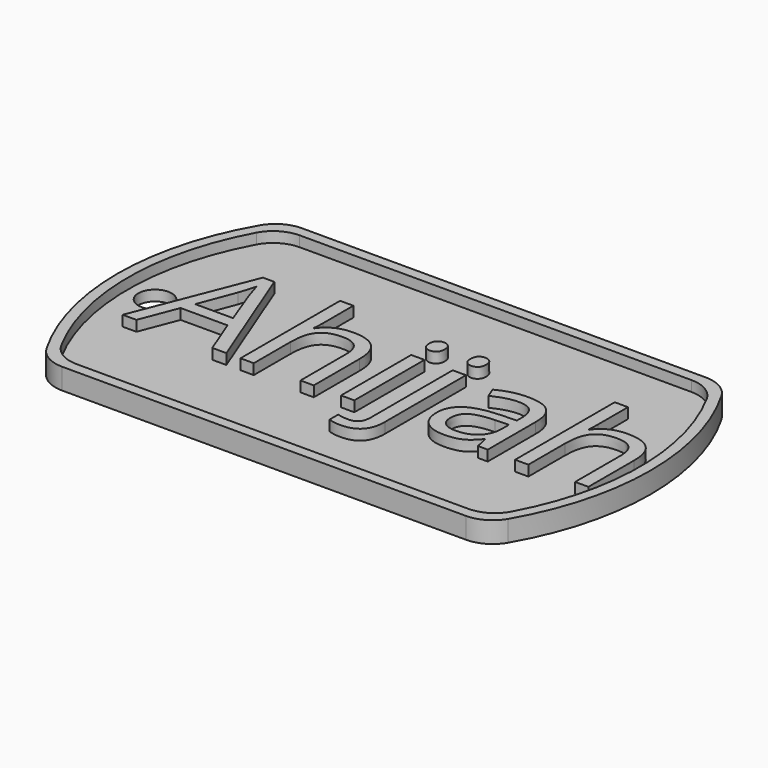
from build123d import *

# Parameters (mm, degrees)
F1_DEPTH     = 1
F3_DEPTH     = 1
F4_R         = 1.5875
F5_DEPTH     = 1
F6_TEXT_SIZE = 15.6169550286
F7_DEPTH     = 1


# Not quite as in the source:
# - Text() gives the source's letters only with a copy of the font that has no kerning and outlines rounded to 1/6400 em; it was checked with that copy


with BuildPart() as f1:
    # F0 (on Top) → F1 (new body)
    with BuildSketch(Plane.XY):
        with BuildLine():
            ThreePointArc((-19.2474145991, 14.2875), (-20.8349145991, 13.862130657), (-21.9970452561, 12.7))
            ThreePointArc((-21.9970452561, 12.7), (-25.4, 0), (-21.9970452561, -12.7))
            ThreePointArc((-21.9970452561, -12.7), (-20.8349145991, -13.862130657), (-19.2474145991, -14.2875))
            Line((-19.2474145991, -14.2875), (19.2474145991, -14.2875))
            ThreePointArc((19.2474145991, -14.2875), (20.8349145991, -13.862130657), (21.9970452561, -12.7))
            ThreePointArc((21.9970452561, -12.7), (25.4, 0), (21.9970452561, 12.7))
            ThreePointArc((21.9970452561, 12.7), (20.8349145991, 13.862130657), (19.2474145991, 14.2875))
            Line((19.2474145991, 14.2875), (-19.2474145991, 14.2875))
        make_face()
    extrude(amount=F1_DEPTH)

    # F2 (on face) → F3 (join)
    with BuildSketch(Plane.XY.offset(1)):
        with BuildLine():
            Line((19.2474145991, 14.2875), (-19.2474145991, 14.2875))
            ThreePointArc((-19.2474145991, 14.2875), (-20.8349145991, 13.862130657), (-21.9970452561, 12.7))
            ThreePointArc((-21.9970452561, 12.7), (-25.4, 0), (-21.9970452561, -12.7))
            ThreePointArc((-21.9970452561, -12.7), (-20.8349145991, -13.862130657), (-19.2474145991, -14.2875))
            Line((-19.2474145991, -14.2875), (19.2474145991, -14.2875))
            ThreePointArc((19.2474145991, -14.2875), (20.8349145991, -13.862130657), (21.9970452561, -12.7))
            ThreePointArc((21.9970452561, -12.7), (25.4, 0), (21.9970452561, 12.7))
            ThreePointArc((21.9970452561, 12.7), (20.8349145991, 13.862130657), (19.2474145991, 14.2875))
        make_face()
        with BuildLine():
            ThreePointArc((-21.4526124879, 11.6252061249), (-20.2856017842, 12.8404540819), (-18.6611352482, 13.2875))
            Line((-18.6611352482, 13.2875), (18.6611352482, 13.2875))
            ThreePointArc((18.6611352482, 13.2875), (20.2856017842, 12.8404540819), (21.4526124879, 11.6252061249))
            ThreePointArc((21.4526124879, 11.6252061249), (24.4, 0), (21.4526124879, -11.6252061249))
            ThreePointArc((21.4526124879, -11.6252061249), (20.2856017842, -12.8404540819), (18.6611352482, -13.2875))
            Line((18.6611352482, -13.2875), (-18.6611352482, -13.2875))
            ThreePointArc((-18.6611352482, -13.2875), (-20.2856017842, -12.8404540819), (-21.4526124879, -11.6252061249))
            ThreePointArc((-21.4526124879, -11.6252061249), (-24.4, 0), (-21.4526124879, 11.6252061249))
        make_face(mode=Mode.SUBTRACT)
    extrude(amount=F3_DEPTH)

    # F4 (on face) → F5 (cut)
    with BuildSketch(Plane.XY.offset(1)):
        with Locations((-21.821282804, 0)):
            Circle(F4_R)
    extrude(amount=-F5_DEPTH, mode=Mode.SUBTRACT)

    # F6 (on face) → F7 (join)
    with BuildSketch(Plane.XY.offset(1)):
        with Locations((-20.9534056485, -4.9375841627)):
            Text('Ahijah', F6_TEXT_SIZE, font='Open Sans', text_align=(TextAlign.LEFT, TextAlign.BOTTOM))
    extrude(amount=F7_DEPTH)


solid = f1.part
